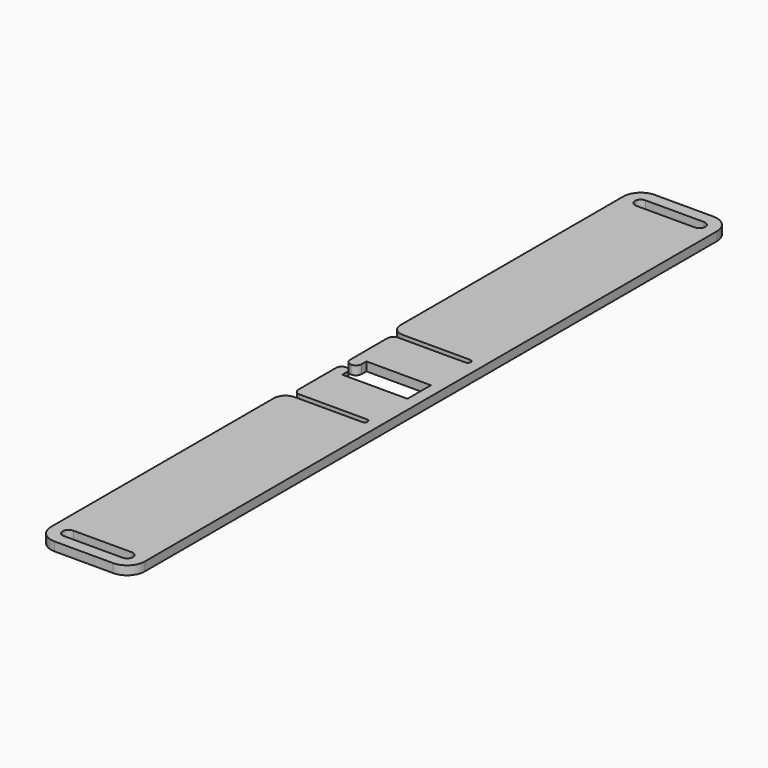
from build123d import *

# Parameters (mm, degrees)
F1_DEPTH    = 1.5
F2_T1_DEPTH = 6.5
F2_T3_DEPTH = 6.4616050658
F3_R        = 2
F4_R        = 3


# Not quite as in the source:
# - a fillet or chamfer that OpenCascade refuses, or shapes differently, is made with other operations: its cross-section is extruded or revolved along the edge and cut away or added


with BuildPart() as f1:
    # F0 (on Top) → F1 (new body)
    with BuildSketch(Plane.XY):
        with BuildLine():
            Line((6.7359172925, 27.2759429877), (-4.7640827075, 27.2759429877))
            ThreePointArc((-4.7640827075, 27.2759429877), (-5.4711894887, 26.9830497689), (-5.7640827075, 26.2759429877))
            Line((-5.7640827075, 26.2759429877), (-5.7640827075, 18.2759429877))
            ThreePointArc((-5.7640827075, 18.2759429877), (-5.4711894887, 17.5688362065), (-4.7640827075, 17.2759429877))
            Line((-4.7640827075, 17.2759429877), (-3.7640827075, 17.2759429877))
            Line((-3.7640827075, 17.2759429877), (-3.7640827075, 19.2759429877))
            Line((-3.7640827075, 19.2759429877), (7.2359172925, 19.2759429877))
            Line((7.2359172925, 19.2759429877), (7.2359172925, 17.2759429877))
            Line((7.2359172925, 17.2759429877), (7.2359172925, 16.2759429877))
            Line((7.2359172925, 16.2759429877), (7.2359172925, 14.2759429877))
            Line((7.2359172925, 14.2759429877), (-3.8877718616, 14.2759429877))
            Line((-3.8877718616, 14.2759429877), (-3.8877718616, 16.2759429877))
            Line((-3.8877718616, 16.2759429877), (-4.7640827075, 16.2759429877))
            ThreePointArc((-4.7640827075, 16.2759429877), (-5.4711894887, 15.9830497689), (-5.7640827075, 15.2759429877))
            Line((-5.7640827075, 15.2759429877), (-5.7640827075, 7.2759429877))
            ThreePointArc((-5.7640827075, 7.2759429877), (-5.4711894887, 6.5688362065), (-4.7640827075, 6.2759429877))
            Line((-4.7640827075, 6.2759429877), (6.7359172925, 6.2759429877))
            ThreePointArc((6.7359172925, 6.2759429877), (7.0894706831, 6.1294963783), (7.2359172925, 5.7759429877))
            ThreePointArc((7.2359172925, 5.7759429877), (7.0894706831, 5.4223895971), (6.7359172925, 5.2759429877))
            Line((6.7359172925, 5.2759429877), (-5.7640827075, 5.2759429877))
            Line((-5.7640827075, 5.2759429877), (-6.7640827075, 5.2759429877))
            Line((-6.7640827075, 5.2759429877), (-6.7640827075, -47.2240570123))
            Line((-6.7640827075, -47.2240570123), (9.2359172925, -47.2240570123))
            Line((9.2359172925, -47.2240570123), (9.2359172925, 80.7759429877))
            Line((9.2359172925, 80.7759429877), (-6.7640827075, 80.7759429877))
            Line((-6.7640827075, 80.7759429877), (-6.7640827075, 28.2759429877))
            Line((-6.7640827075, 28.2759429877), (-5.7640827075, 28.2759429877))
            Line((-5.7640827075, 28.2759429877), (6.7359172925, 28.2759429877))
            ThreePointArc((6.7359172925, 28.2759429877), (7.0894706831, 28.1294963783), (7.2359172925, 27.7759429877))
            ThreePointArc((7.2359172925, 27.7759429877), (7.0894706831, 27.4223895971), (6.7359172925, 27.2759429877))
        make_face()
        with BuildLine():
            ThreePointArc((-4.7640827075, -44.2240570123), (-4.4711894887, -43.5169502311), (-3.7640827075, -43.2240570123))
            Line((-3.7640827075, -43.2240570123), (6.2359172925, -43.2240570123))
            ThreePointArc((6.2359172925, -43.2240570123), (6.9430240737, -43.5169502311), (7.2359172925, -44.2240570123))
            ThreePointArc((7.2359172925, -44.2240570123), (6.9430240737, -44.9311637935), (6.2359172925, -45.2240570123))
            Line((6.2359172925, -45.2240570123), (-3.7640827075, -45.2240570123))
            ThreePointArc((-3.7640827075, -45.2240570123), (-4.4711894887, -44.9311637935), (-4.7640827075, -44.2240570123))
        make_face(mode=Mode.SUBTRACT)
        with BuildLine():
            Line((6.2359172925, 76.7759429877), (-3.7640827075, 76.7759429877))
            ThreePointArc((-3.7640827075, 76.7759429877), (-4.4711894887, 77.0688362065), (-4.7640827075, 77.7759429877))
            ThreePointArc((-4.7640827075, 77.7759429877), (-4.4711894887, 78.4830497689), (-3.7640827075, 78.7759429877))
            Line((-3.7640827075, 78.7759429877), (6.2359172925, 78.7759429877))
            ThreePointArc((6.2359172925, 78.7759429877), (6.9430240737, 78.4830497689), (7.2359172925, 77.7759429877))
            ThreePointArc((7.2359172925, 77.7759429877), (6.9430240737, 77.0688362065), (6.2359172925, 76.7759429877))
        make_face(mode=Mode.SUBTRACT)
    extrude(amount=F1_DEPTH)

    # F2: fillet of radius 1 on 2 edges, made by hand

    # F2_s2 → F2_t1 (cut)
    with BuildSketch(Plane.XY.offset(-2.5)):
        with BuildLine():
            ThreePointArc((-3.7640827075, 18.2759429877), (-4.0569759263, 17.5688362065), (-4.7640827075, 17.2759429877))
            Line((-4.7640827075, 17.2759429877), (-3.7640827075, 17.2759429877))
            Line((-3.7640827075, 17.2759429877), (-3.7640827075, 18.2759429877))
        make_face()
    extrude(amount=F2_T1_DEPTH, mode=Mode.SUBTRACT)

    # F2_s4 → F2_t3 (cut)
    with BuildSketch(Plane.XY.offset(-2.4808025329)):
        with BuildLine():
            ThreePointArc((-4.7640827075, 16.2759429877), (-4.1382089376, 15.94555507), (-3.8877718616, 15.2836219745))
            Line((-3.8877718616, 15.2836219745), (-3.8877718616, 16.2759429877))
            Line((-3.8877718616, 16.2759429877), (-4.7640827075, 16.2759429877))
        make_face()
    extrude(amount=F2_T3_DEPTH, mode=Mode.SUBTRACT)

    # F3
    f3_edges = [f1.edges().sort_by_distance(p)[0] for p in [
        (-6.764083, 28.275943, 0.75),
        (-6.764083, 5.275943, 0.75),
    ]]
    fillet(f3_edges, radius=F3_R)

    # F4
    f4_edges = [f1.edges().sort_by_distance(p)[0] for p in [
        (9.235917, 80.775943, 0.75),
        (-6.764083, 80.775943, 0.75),
        (-6.764083, -47.224057, 0.75),
        (9.235917, -47.224057, 0.75),
    ]]
    fillet(f4_edges, radius=F4_R)


solid = f1.part
